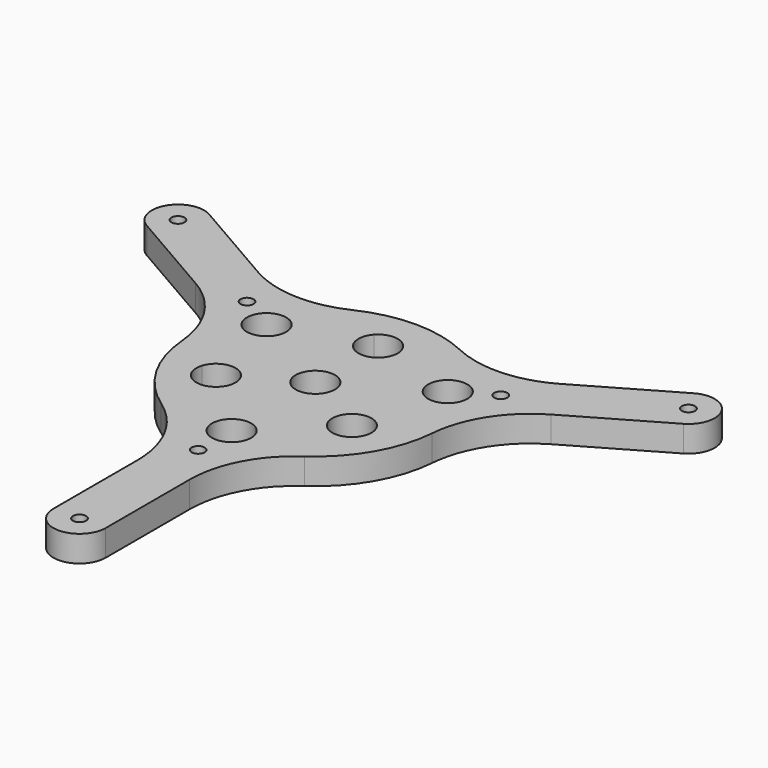
from build123d import *

# Parameters (mm, degrees)
F0_R        = 1.5875
F0_R_2      = 4.7625
F1_DEPTH    = 6.35
F2_T1_DEPTH = 6.35
F3_R        = 25.6632962838


# Not quite as in the source:
# - a fillet or chamfer that OpenCascade refuses, or shapes differently, is made with other operations: its cross-section is extruded or revolved along the edge and cut away or added
# - a length typed as a fraction of an inch, garbled in the dataset ("3 / 203.2 mm" for 3/8 in), is restored


with BuildPart() as f1:
    # F0 (on Top) → F1 (new body)
    with BuildSketch(Plane.XY):
        with BuildLine():
            Line((25.7948291982, 22.225), (38.4948291982, 22.225))
            Line((38.4948291982, 22.225), (32.1448291982, 11.2264773719))
            Line((32.1448291982, 11.2264773719), (65.1403970824, 30.2764773719))
            ThreePointArc((65.1403970824, 30.2764773719), (67.4646583964, 38.950738686), (58.7903970824, 41.275))
            Line((58.7903970824, 41.275), (25.7948291982, 22.225))
        make_face()
        with Locations((61.9653970824, 35.775738686)):
            Circle(F0_R, mode=Mode.SUBTRACT)
        with BuildLine():
            Line((32.1448291982, 11.2264773719), (38.4948291982, 22.225))
            Line((38.4948291982, 22.225), (25.7948291982, 22.225))
            Line((25.7948291982, 22.225), (20.8585659862, 22.225))
            ThreePointArc((20.8585659862, 22.225), (26.3964543073, 15.24), (29.6766975922, 6.9515480306))
            Line((29.6766975922, 6.9515480306), (32.1448291982, 11.2264773719))
        make_face()
        with Locations((30.7958633586, 17.78)):
            Circle(F0_R, mode=Mode.SUBTRACT)
        with BuildLine():
            ThreePointArc((30.48, 0), (30.2785084062, 3.4989039276), (29.6766975922, 6.9515480306))
            Line((29.6766975922, 6.9515480306), (21.0222935562, -8.0383194689))
            ThreePointArc((21.0222935562, -8.0383194689), (21.2004099791, -8.7721955059), (21.2602839421, -9.525))
            ThreePointArc((21.2602839421, -9.525), (20.1939753076, -12.5282608344), (17.472535642, -14.1866805311))
            Line((17.472535642, -14.1866805311), (8.818131606, -29.1765480305))
            ThreePointArc((8.818131606, -29.1765480305), (24.4725055047, -18.1693938898), (30.48, 0))
        make_face()
        with BuildLine():
            Line((21.0222935562, -8.0383194689), (29.6766975922, 6.9515480306))
            ThreePointArc((29.6766975922, 6.9515480306), (26.3964543073, 15.24), (20.8585659862, 22.225))
            Line((20.8585659862, 22.225), (3.5497579143, 22.225))
            ThreePointArc((3.5497579143, 22.225), (4.4489958596, 20.7493652025), (4.7625, 19.05))
            ThreePointArc((4.7625, 19.05), (-1.6993652025, 14.6010041404), (-3.5497579143, 22.225))
            Line((-3.5497579143, 22.225), (-20.8585659862, 22.225))
            ThreePointArc((-20.8585659862, 22.225), (-26.3964543073, 15.24), (-29.6766975922, 6.9515480306))
            Line((-29.6766975922, 6.9515480306), (-21.0222935562, -8.0383194689))
            ThreePointArc((-21.0222935562, -8.0383194689), (-15.744979448, -4.822373963), (-11.7352839421, -9.525))
            ThreePointArc((-11.7352839421, -9.525), (-13.4945231077, -13.2211913655), (-17.472535642, -14.1866805311))
            Line((-17.472535642, -14.1866805311), (-8.818131606, -29.1765480305))
            ThreePointArc((-8.818131606, -29.1765480305), (0, -30.48), (8.818131606, -29.1765480305))
            Line((8.818131606, -29.1765480305), (17.472535642, -14.1866805311))
            ThreePointArc((17.472535642, -14.1866805311), (12.3733379566, -7.14375), (21.0222935562, -8.0383194689))
        make_face()
        with Locations((0, -25.4)):
            Circle(F0_R_2, mode=Mode.SUBTRACT)
        with Locations((-21.9970452561, 12.7)):
            Circle(F0_R_2, mode=Mode.SUBTRACT)
        Circle(F0_R_2, mode=Mode.SUBTRACT)
        with Locations((21.9970452561, 12.7)):
            Circle(F0_R_2, mode=Mode.SUBTRACT)
        with BuildLine():
            Line((3.5497579143, 22.225), (20.8585659862, 22.225))
            ThreePointArc((20.8585659862, 22.225), (0, 30.48), (-20.8585659862, 22.225))
            Line((-20.8585659862, 22.225), (-3.5497579143, 22.225))
            ThreePointArc((-3.5497579143, 22.225), (0, 23.8125), (3.5497579143, 22.225))
        make_face()
        with BuildLine():
            ThreePointArc((-29.6766975922, 6.9515480306), (-26.3964543073, 15.24), (-20.8585659862, 22.225))
            Line((-20.8585659862, 22.225), (-25.7948291982, 22.225))
            Line((-25.7948291982, 22.225), (-38.4948291982, 22.225))
            Line((-38.4948291982, 22.225), (-32.1448291982, 11.2264773719))
            Line((-32.1448291982, 11.2264773719), (-29.6766975922, 6.9515480306))
        make_face()
        with Locations((-30.7958633586, 17.78)):
            Circle(F0_R, mode=Mode.SUBTRACT)
        with BuildLine():
            Line((6.35, -33.4514773719), (8.818131606, -29.1765480305))
            ThreePointArc((8.818131606, -29.1765480305), (0, -30.48), (-8.818131606, -29.1765480305))
            Line((-8.818131606, -29.1765480305), (-6.35, -33.4514773719))
            Line((-6.35, -33.4514773719), (0, -44.45))
            Line((0, -44.45), (6.35, -33.4514773719))
        make_face()
        with Locations((0, -35.56)):
            Circle(F0_R, mode=Mode.SUBTRACT)
        with BuildLine():
            Line((-38.4948291982, 22.225), (-25.7948291982, 22.225))
            Line((-25.7948291982, 22.225), (-58.7903970824, 41.275))
            ThreePointArc((-58.7903970824, 41.275), (-67.4646583964, 38.950738686), (-65.1403970824, 30.2764773719))
            Line((-65.1403970824, 30.2764773719), (-32.1448291982, 11.2264773719))
            Line((-32.1448291982, 11.2264773719), (-38.4948291982, 22.225))
        make_face()
        with Locations((-61.9653970824, 35.775738686)):
            Circle(F0_R, mode=Mode.SUBTRACT)
        with BuildLine():
            Line((-21.0222935562, -8.0383194689), (-29.6766975922, 6.9515480306))
            ThreePointArc((-29.6766975922, 6.9515480306), (-26.3964543073, -15.24), (-8.818131606, -29.1765480305))
            Line((-8.818131606, -29.1765480305), (-17.472535642, -14.1866805311))
            ThreePointArc((-17.472535642, -14.1866805311), (-20.6222299276, -11.90625), (-21.0222935562, -8.0383194689))
        make_face()
        with BuildLine():
            Line((6.35, -71.5514773719), (6.35, -33.4514773719))
            Line((6.35, -33.4514773719), (0, -44.45))
            Line((0, -44.45), (-6.35, -33.4514773719))
            Line((-6.35, -33.4514773719), (-6.35, -71.5514773719))
            ThreePointArc((-6.35, -71.5514773719), (0, -77.9014773719), (6.35, -71.5514773719))
        make_face()
        with Locations((0, -71.5514773719)):
            Circle(F0_R, mode=Mode.SUBTRACT)
    extrude(amount=F1_DEPTH)

    # F2: fillet of radius 50.8 on 6 edges, made by hand

    # F2_s2 → F2_t1 (join)
    with BuildSketch(Plane.XY):
        with BuildLine():
            ThreePointArc((29.6766975922, 6.9515480306), (35.4424077678, 12.4134665997), (41.9889550232, 16.9099860669))
            Line((41.9889550232, 16.9099860669), (32.1448291982, 11.2264773719))
            Line((32.1448291982, 11.2264773719), (29.6766975922, 6.9515480306))
        make_face()
        with BuildLine():
            ThreePointArc((35.6389550232, 27.908508695), (28.4715813083, 24.4872921983), (20.8585659862, 22.225))
            Line((20.8585659862, 22.225), (25.7948291982, 22.225))
            Line((25.7948291982, 22.225), (35.6389550232, 27.908508695))
        make_face()
        with BuildLine():
            ThreePointArc((-20.8585659862, 22.225), (-28.4715813083, 24.4872921983), (-35.6389550232, 27.908508695))
            Line((-35.6389550232, 27.908508695), (-25.7948291982, 22.225))
            Line((-25.7948291982, 22.225), (-20.8585659862, 22.225))
        make_face()
        with BuildLine():
            ThreePointArc((-41.9889550232, 16.9099860669), (-35.4424077678, 12.4134665997), (-29.6766975922, 6.9515480306))
            Line((-29.6766975922, 6.9515480306), (-32.1448291982, 11.2264773719))
            Line((-32.1448291982, 11.2264773719), (-41.9889550232, 16.9099860669))
        make_face()
        with BuildLine():
            ThreePointArc((-8.818131606, -29.1765480305), (-6.9708264595, -36.9007587981), (-6.35, -44.8184947619))
            Line((-6.35, -44.8184947619), (-6.35, -33.4514773719))
            Line((-6.35, -33.4514773719), (-8.818131606, -29.1765480305))
        make_face()
        with BuildLine():
            ThreePointArc((6.35, -44.8184947619), (6.9708264595, -36.9007587981), (8.818131606, -29.1765480305))
            Line((8.818131606, -29.1765480305), (6.35, -33.4514773719))
            Line((6.35, -33.4514773719), (6.35, -44.8184947619))
        make_face()
    extrude(amount=F2_T1_DEPTH)

    # F3
    f3_edges = [f1.edges().sort_by_distance(p)[0] for p in [
        (-29.676698, 6.951548, 3.175),
        (-8.818132, -29.176548, 3.175),
        (8.818132, -29.176548, 3.175),
        (29.676698, 6.951548, 3.175),
        (20.858566, 22.225, 3.175),
        (-20.858566, 22.225, 3.175),
    ]]
    fillet(f3_edges, radius=F3_R)


solid = f1.part
